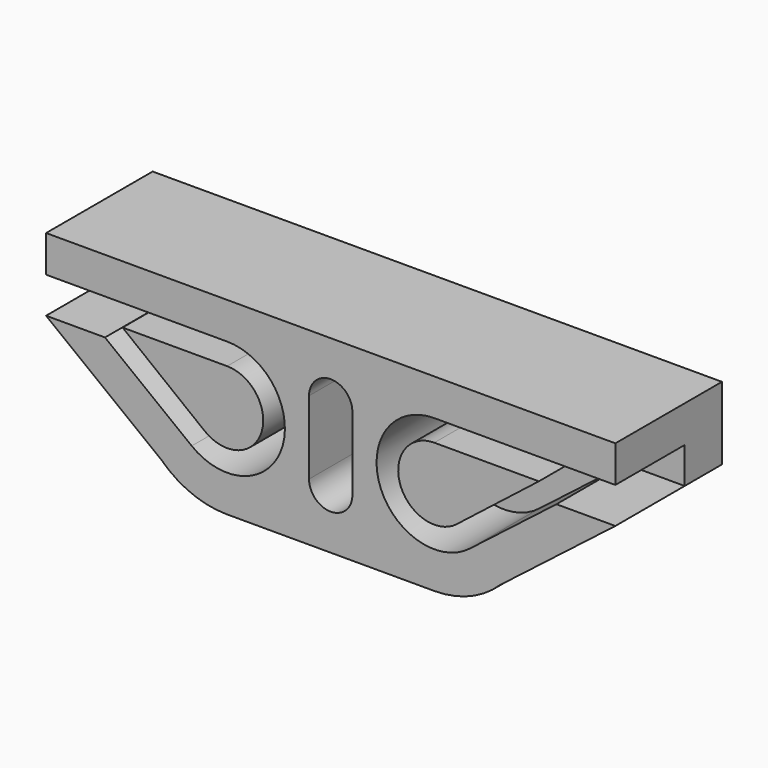
from build123d import *

# Parameters (mm, degrees)
F2_DEPTH  = 8
F3_W      = 40
F3_H      = 13.08
F4_DEPTH  = 2
F8_DEPTH  = 25.4
F9_DEPTH  = 0.2869853
F10_DEPTH = 0.2869852618
F11_DEPTH = 1.225
F13_DEPTH = 25.4


# Not quite as in the source:
# - an extrude ends at something that could not be found from the text; its depth is read off the source's solid


with BuildPart() as f2:
    # F1 (on Front) → F2 (new body)
    with BuildSketch(Plane.XZ):
        with BuildLine():
            Line((0, -2.26), (-20, -2.26))
            Line((-20, -2.26), (-20, -4.8))
            Line((-20, -4.8), (-7.175, -4.8))
            ThreePointArc((-7.175, -4.8), (-3.3907124319, -10.0958269953), (-9.6268909943, -11.9604161992))
            Line((-9.6268909943, -11.9604161992), (-15.6340319663, -7.3))
            Line((-15.6340319663, -7.3), (-20, -7.3))
            Line((-20, -7.3), (-20, -15.34))
            Line((-20, -15.34), (0, -15.34))
            Line((0, -15.34), (20, -15.34))
            Line((20, -15.34), (20, -7.3))
            Line((20, -7.3), (15.6340319663, -7.3))
            Line((15.6340319663, -7.3), (9.6268909943, -11.9604161992))
            ThreePointArc((9.6268909943, -11.9604161992), (3.3907124319, -10.0958269953), (7.175, -4.8))
            Line((7.175, -4.8), (20, -4.8))
            Line((20, -4.8), (20, -2.26))
            Line((20, -2.26), (0, -2.26))
        make_face()
    extrude(amount=F2_DEPTH)


with BuildPart() as f2b:
    # F1 (on Front) → F2, piece 2 (new body)
    with BuildSketch(Plane.XZ):
        with BuildLine():
            Line((-14.4153116271, -6.3), (-8.7175368467, -10.7673789865))
            ThreePointArc((-8.7175368467, -10.7673789865), (-4.8119037825, -9.6159511424), (-7.175, -6.3))
            Line((-7.175, -6.3), (-14.4153116271, -6.3))
        make_face()
    extrude(amount=F2_DEPTH)


with BuildPart() as f2c:
    # F1 (on Front) → F2, piece 3 (new body)
    with BuildSketch(Plane.XZ):
        with BuildLine():
            Line((8.7175368467, -10.7673789865), (14.4153116271, -6.3))
            Line((14.4153116271, -6.3), (7.175, -6.3))
            ThreePointArc((7.175, -6.3), (4.8119037825, -9.6159511424), (8.7175368467, -10.7673789865))
        make_face()
    extrude(amount=F2_DEPTH)


with BuildPart() as f4:
    # F3 (on face) → F4 (new body)
    with BuildSketch(Plane(origin=(0, 0, 0), x_dir=(-1, 0, 0), z_dir=(0, 1, 0))):
        with Locations((0, -8.8)):
            Rectangle(F3_W, F3_H)
    extrude(amount=-F4_DEPTH)

    # F5: union F2
    add(f2.part)


with BuildPart() as f2c_1:
    add(f2c.part)

    # F6: union F4, F2b
    add(f4.part)
    add(f2b.part)

    # F7 (on face) → F8 (cut)
    with BuildSketch(Plane.XZ.offset(8)):
        with BuildLine():
            Line((22.5005224347, -7.3), (20, -7.3))
            Line((20, -7.3), (19.7130147382, -7.3))
            Line((19.7130147382, -7.3), (11.7279629554, -13.4949045067))
            ThreePointArc((11.7279629554, -13.4949045067), (9.6313107017, -14.8611993646), (7.175, -15.34))
            Line((7.175, -15.34), (7.175, -19.2080270499))
            Line((7.175, -19.2080270499), (22.5005224347, -19.2080270499))
            Line((22.5005224347, -19.2080270499), (22.5005224347, -7.3))
        make_face()
        with BuildLine():
            Line((-19.7130147382, -7.3), (-20, -7.3))
            Line((-20, -7.3), (-22.5005224347, -7.3))
            Line((-22.5005224347, -7.3), (-22.5005224347, -19.2080270499))
            Line((-22.5005224347, -19.2080270499), (-7.175, -19.2080270499))
            Line((-7.175, -19.2080270499), (-7.175, -15.34))
            ThreePointArc((-7.175, -15.34), (-9.6313107017, -14.8611993646), (-11.7279629554, -13.4949045067))
            Line((-11.7279629554, -13.4949045067), (-19.7130147382, -7.3))
        make_face()
    extrude(amount=-F8_DEPTH, mode=Mode.SUBTRACT)

    # F9 (cut, through all): a face of the model
    f9_faces = [f2c_1.faces().sort_by_distance(p)[0] for p in [
        (20, -3.4075829384, -4.0276303318),
    ]]
    extrude(f9_faces, amount=-F9_DEPTH, mode=Mode.SUBTRACT)

    # F10 (cut, through all): a face of the model
    f10_faces = [f2c_1.faces().sort_by_distance(p)[0] for p in [
        (-20, -3.4075829384, -4.0276303318),
    ]]
    extrude(f10_faces, amount=-F10_DEPTH, mode=Mode.SUBTRACT)

    # F11 (add): a face of the model
    f11_faces = [f2c_1.faces().sort_by_distance(p)[0] for p in [
        (-8.8e-09, 0, -8.042025569),
    ]]
    extrude(f11_faces, amount=F11_DEPTH)

    # F12 (on face) → F13 (cut)
    with BuildSketch(Plane.XZ.offset(8)):
        with BuildLine():
            ThreePointArc((-1.5, -11.34), (0, -12.84), (1.5, -11.34))
            Line((1.5, -11.34), (1.5, -6.26))
            ThreePointArc((1.5, -6.26), (0, -4.76), (-1.5, -6.26))
            Line((-1.5, -6.26), (-1.5, -11.34))
        make_face()
    extrude(amount=-F13_DEPTH, mode=Mode.SUBTRACT)


solid = f2c_1.part
